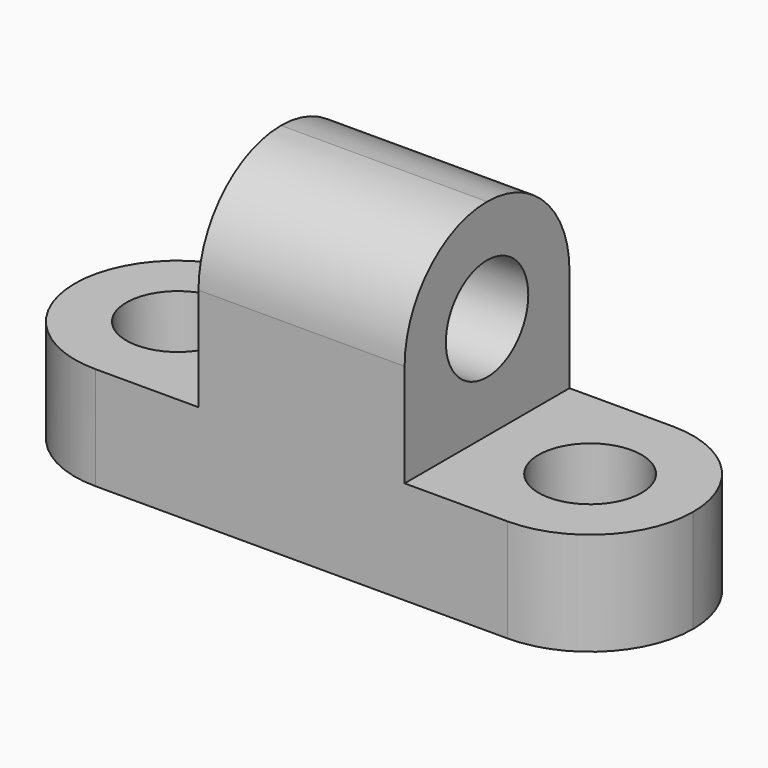
from build123d import *

# Parameters (mm, degrees)
F1_DEPTH  = 25.4
F2_R      = 12.7
F3_R      = 12.69999
F4_R      = 12.7
F5_R      = 12.69999
F6_R      = 12.7
F7_R      = 12.69999
F8_R      = 6.35
F9_DEPTH  = 25.4
F10_R     = 6.35
F11_DEPTH = 25.4
F12_R     = 6.35
F13_DEPTH = 25.4


# Not quite as in the source:
# - a fillet or chamfer is up to 0.001 mm smaller than in the source, because OpenCascade refuses the exact size


with BuildPart() as f1:
    # F0 (on Front) → F1 (new body)
    with BuildSketch(Plane.XZ):
        Polygon((0, 12.7), (0, 0), (76.2, 0), (76.2, 12.7), (50.8, 12.7), (50.8, 38.1), (25.4, 38.1), (25.4, 12.7), align=None)
    extrude(amount=F1_DEPTH)

    # F2
    f2_edges = [f1.edges().sort_by_distance(p)[0] for p in [
        (76.2, -25.4, 6.35),
    ]]
    fillet(f2_edges, radius=F2_R)

    # F3 (radius 12.7 in the source; OpenCascade refuses exactly that, so slightly less here)
    f3_edges = [f1.edges().sort_by_distance(p)[0] for p in [
        (76.2, 0, 6.35),
    ]]
    fillet(f3_edges, radius=F3_R)

    # F4
    f4_edges = [f1.edges().sort_by_distance(p)[0] for p in [
        (0, -25.4, 6.35),
    ]]
    fillet(f4_edges, radius=F4_R)

    # F5 (radius 12.7 in the source; OpenCascade refuses exactly that, so slightly less here)
    f5_edges = [f1.edges().sort_by_distance(p)[0] for p in [
        (0, 0, 6.35),
    ]]
    fillet(f5_edges, radius=F5_R)

    # F6
    f6_edges = [f1.edges().sort_by_distance(p)[0] for p in [
        (38.1, 0, 38.1),
    ]]
    fillet(f6_edges, radius=F6_R)

    # F7 (radius 12.7 in the source; OpenCascade refuses exactly that, so slightly less here)
    f7_edges = [f1.edges().sort_by_distance(p)[0] for p in [
        (38.1, -25.4, 38.1),
    ]]
    fillet(f7_edges, radius=F7_R)

    # F8 (on face) → F9 (cut)
    with BuildSketch(Plane.YZ.offset(50.8)):
        with Locations((-12.7, 25.4)):
            Circle(F8_R)
    extrude(amount=-F9_DEPTH, mode=Mode.SUBTRACT)

    # F10 (on face) → F11 (cut)
    with BuildSketch(Plane.XY.offset(12.7)):
        with Locations((63.5, -12.7)):
            Circle(F10_R)
    extrude(amount=-F11_DEPTH, mode=Mode.SUBTRACT)

    # F12 (on face) → F13 (cut)
    with BuildSketch(Plane.XY.offset(12.7)):
        with Locations((12.7, -12.7)):
            Circle(F12_R)
    extrude(amount=-F13_DEPTH, mode=Mode.SUBTRACT)


solid = f1.part
